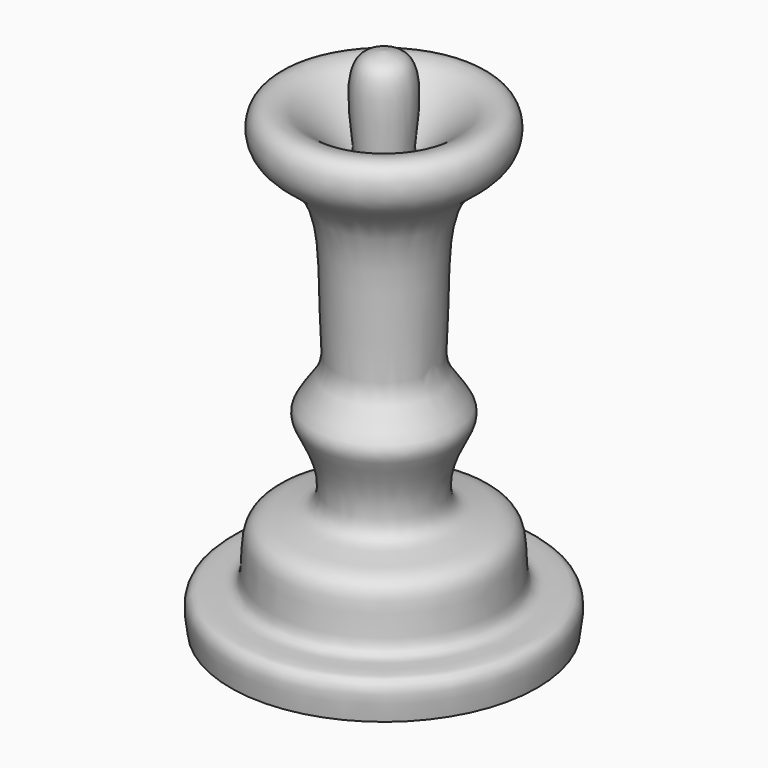
from build123d import *


with BuildPart() as f1:
    # F0 (on Front) → F1 (revolve)
    with BuildSketch(Plane.XZ):
        with BuildLine():
            Line((9.6333737232, -22.384019196), (24.6333737232, -22.384019196))
            add(Edge.make_bspline(
                [(9.6333737232, 27.615980804), (10.4218008869, 27.5161598405), (12.3862150538, 27.2674498469), (12.4957704572, 22.2732189561), (11.3582118021, 16.6759341753), (16.5116833203, 23.3477614616), (20.3341286803, 23.1335308453), (20.4371584929, 18.4835693412), (14.2307797327, 16.3198087464), (14.8565541303, 4.9231923709), (13.89984472, 0.068755464), (17.6420746833, -3.2103347088), (15.2731452635, -6.0750096953), (13.6981431476, -12.9169973259), (21.7654394003, -11.5217330985), (19.4724426724, -19.7783412981), (25.3624751165, -17.8291953544), (24.8785161083, -20.8525718685), (24.6333737232, -22.384019196)],
                knots=[0, 0, 0, 0, 0.0444048583, 0.1106374015, 0.1639043912, 0.2363941814, 0.2877235313, 0.3409905211, 0.4107938409, 0.507756539, 0.5745080538, 0.6321783663, 0.6870682269, 0.7546297819, 0.8211432996, 0.8893369144, 0.9439452262, 1, 1, 1, 1], degree=3))
            Line((9.6333737232, 27.615980804), (9.6333737232, -22.384019196))
        make_face()
    revolve(axis=Axis((9.6333737232, 0, 2.615980804), (0, 0, 1)))


solid = f1.part
